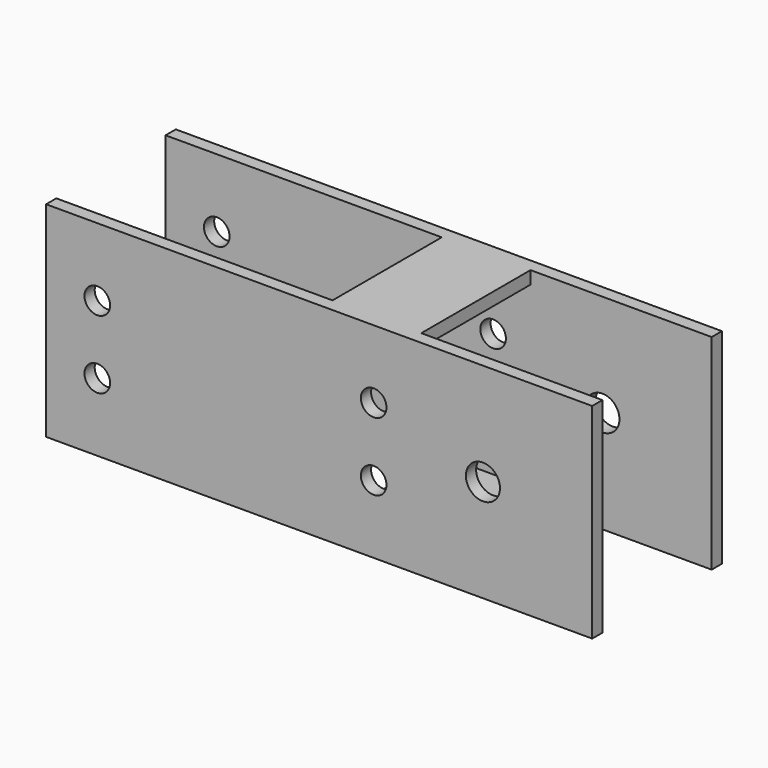
from build123d import *

# Parameters (mm, degrees)
F0_W     = 203.2
F0_H     = 76.2
F0_R     = 4.7625
F0_R_2   = 6.35
F1_DEPTH = 60.325
F3_W     = 102.7627293737
F3_H     = 50.8
F4_DEPTH = 85.725
F5_W     = 50.8
F5_H     = 66.675
F6_DEPTH = 203.2
F7_W     = 67.4074530634
F7_H     = 50.8
F8_DEPTH = 76.2


with BuildPart() as f1:
    # F0 (on Front) → F1 (new body)
    with BuildSketch(Plane.XZ):
        with Locations((101.6, 38.1)):
            Rectangle(F0_W, F0_H)
        with Locations((19.05, 25.4)):
            Circle(F0_R, mode=Mode.SUBTRACT)
        with Locations((121.8779161572, 25.4)):
            Circle(F0_R, mode=Mode.SUBTRACT)
        with Locations((19.05, 50.8)):
            Circle(F0_R, mode=Mode.SUBTRACT)
        with Locations((121.8779161572, 50.8)):
            Circle(F0_R, mode=Mode.SUBTRACT)
        with Locations((162.5389580786, 38.1)):
            Circle(F0_R_2, mode=Mode.SUBTRACT)
    extrude(amount=-F1_DEPTH)

    # F3 (on offset) → F4 (cut)
    with BuildSketch(Plane.XY.offset(76.2)):
        with Locations((51.3813646869, 30.1625)):
            Rectangle(F3_W, F3_H)
    extrude(amount=-F4_DEPTH, mode=Mode.SUBTRACT)

    # F5 (on Right) → F6 (cut)
    with BuildSketch(Plane.YZ):
        with Locations((30.1625, 38.1)):
            Rectangle(F5_W, F5_H)
    extrude(amount=F6_DEPTH, mode=Mode.SUBTRACT)

    # F7 (on Top) → F8 (cut)
    with BuildSketch(Plane.XY):
        with Locations((169.4962734683, 30.1625)):
            Rectangle(F7_W, F7_H)
    extrude(amount=F8_DEPTH, mode=Mode.SUBTRACT)


solid = f1.part
